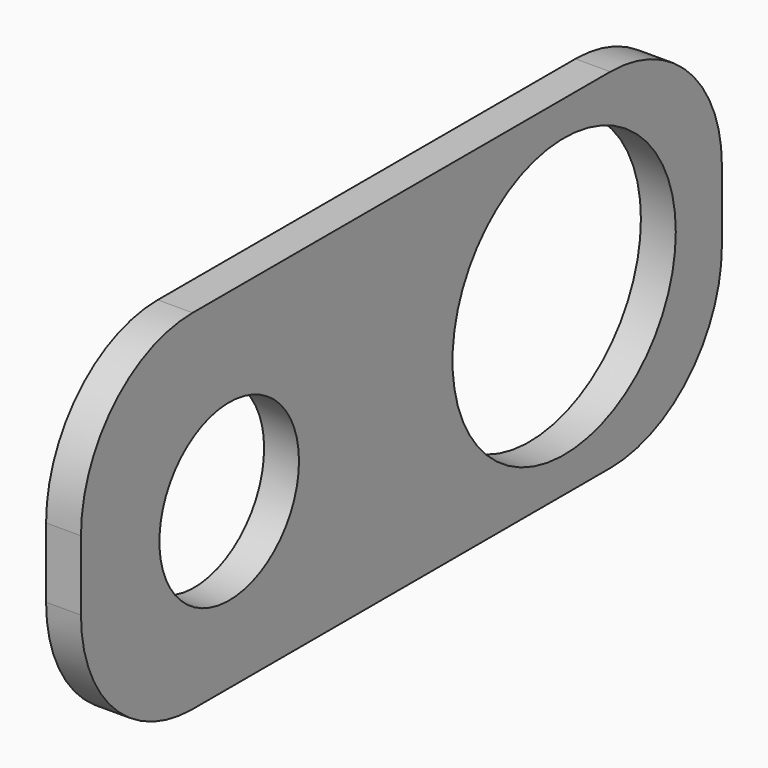
from build123d import *

# Parameters (mm, degrees)
F0_R     = 7.9375
F0_R_2   = 12.7
F1_DEPTH = 3.175


# Not quite as in the source:
# - a length typed as a fraction of an inch, garbled in the dataset ("3 / 203.2 mm" for 3/8 in), is restored


with BuildPart() as f1:
    # F0 (on Right) → F1 (new body)
    with BuildSketch(Plane.YZ):
        with BuildLine():
            Line((35.9976727843, 33.7128622103), (-11.5086332291, 33.7128622103))
            ThreePointArc((-11.5086332291, 33.7128622103), (-20.4888893502, 29.9931183314), (-24.2086332291, 21.0128622103))
            Line((-24.2086332291, 21.0128622103), (-24.2086332291, 14.6628622103))
            ThreePointArc((-24.2086332291, 14.6628622103), (-20.4888893502, 5.6826060893), (-11.5086332291, 1.9628622103))
            Line((-11.5086332291, 1.9628622103), (35.9976727843, 1.9628622103))
            ThreePointArc((35.9976727843, 1.9628622103), (44.9779289054, 5.6826060893), (48.6976727843, 14.6628622103))
            Line((48.6976727843, 14.6628622103), (48.6976727843, 21.0128622103))
            ThreePointArc((48.6976727843, 21.0128622103), (44.9779289054, 29.9931183314), (35.9976727843, 33.7128622103))
        make_face()
        with Locations((-7.3484922707, 16.9180016965)):
            Circle(F0_R, mode=Mode.SUBTRACT)
        with Locations((30.7515077293, 17.8526993841)):
            Circle(F0_R_2, mode=Mode.SUBTRACT)
    extrude(amount=F1_DEPTH)


solid = f1.part
